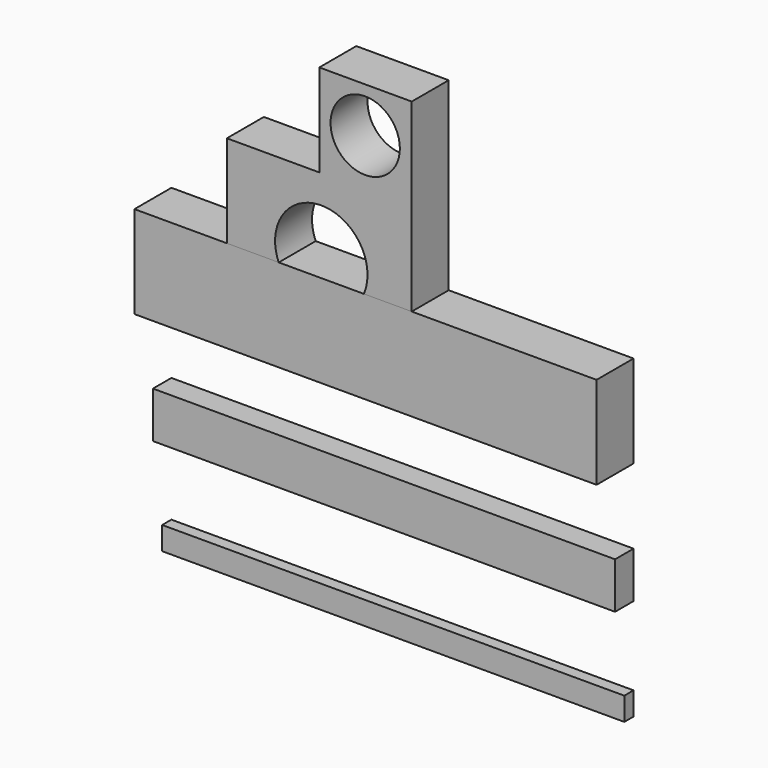
from build123d import *

# Parameters (mm, degrees)
F0_W     = 25.4
F0_H     = 25.4
F1_DEPTH = 12.7
F2_R     = 3.175
F2_R_2   = 6.35
F2_R_3   = 9.525
F2_R_4   = 12.7
F3_DEPTH = 170.688
F4_W     = 127
F4_H     = 25.4
F5_DEPTH = 12.7
F4_H_2   = 12.7
F6_DEPTH = 6.35
F4_H_3   = 6.35
F7_DEPTH = 3.175


# Not quite as in the source:
# - a feature of the source that left no trace in its solid (it failed there, or was rolled back) is left out


with BuildPart() as f1:
    # F0 (on Front) → F1 (new body)
    with BuildSketch(Plane.XZ):
        with Locations((12.7, 12.7)):
            Rectangle(F0_W, F0_H)
        Polygon((25.4, 25.4), (25.4, 0), (50.8, 0), (50.8, 50.8), (25.4, 50.8), align=None)
        Polygon((50.8, 50.8), (50.8, 0), (76.2, 0), (76.2, 76.2), (50.8, 76.2), align=None)
    extrude(amount=F1_DEPTH)

    # F2 (on face) → F3 (cut)
    with BuildSketch(Plane.XZ.offset(12.7)):
        with Locations((12.9853840917, 12.3338634148)):
            Circle(F2_R)
        with Locations((29.6258646995, 13.3764185011)):
            Circle(F2_R_2)
        with Locations((63.4126663208, 63.7898892164)):
            Circle(F2_R_3)
        with Locations((51.3470545411, 30.3075592965)):
            Circle(F2_R_4)
    extrude(amount=-F3_DEPTH, mode=Mode.SUBTRACT)


with BuildPart() as f5:
    # F4 (on Front) → F5 (new body)
    with BuildSketch(Plane.XZ):
        with Locations((63.5, 12.7)):
            Rectangle(F4_W, F4_H)
    extrude(amount=F5_DEPTH)


with BuildPart() as f6:
    # F4 (on Front) → F6 (new body)
    with BuildSketch(Plane.XZ):
        with Locations((63.5, -26.9509138703)):
            Rectangle(F4_W, F4_H_2)
    extrude(amount=F6_DEPTH)


with BuildPart() as f7:
    # F4 (on Front) → F7 (new body)
    with BuildSketch(Plane.XZ):
        with Locations((63.5, -58.057842505)):
            Rectangle(F4_W, F4_H_3)
    extrude(amount=F7_DEPTH)


solid = Compound([f1.part, f5.part, f6.part, f7.part])
